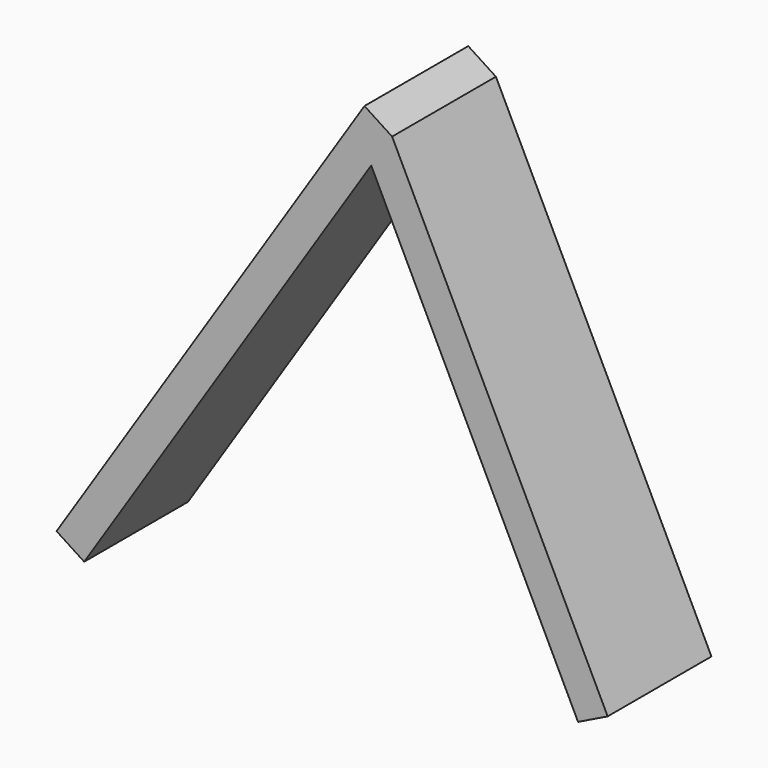
from build123d import *

# Parameters (mm, degrees)
F1_E0_W  = 43.5960156369
F1_E0_H  = 10
F2_DEPTH = 2.54
F1_E1_W  = 37.7890589032
F1_E1_H  = 10
F3_DEPTH = 2.54


with BuildPart() as f2:
    # F1_E0 (on explicit) → F2 (new body)
    with BuildSketch(Plane(origin=(-52.6879653335, 0, -36.5696884692), x_dir=(0.5443919443, 0, 0.8388309788), z_dir=(0.8388309788, 0, -0.5443919443))):
        with Locations((21.7980078184, 5)):
            Rectangle(F1_E0_W, F1_E0_H)
    extrude(amount=-F2_DEPTH)

    # F1_E1 (on explicit) → F3 (join)
    with BuildSketch(Plane(origin=(-28.9546456188, 0, 0), x_dir=(0.4396331317, 0, -0.8981774376), z_dir=(-0.8981774376, 0, -0.4396331317))):
        with Locations((18.8945294516, 5)):
            Rectangle(F1_E1_W, F1_E1_H)
    extrude(amount=F3_DEPTH)


solid = f2.part
